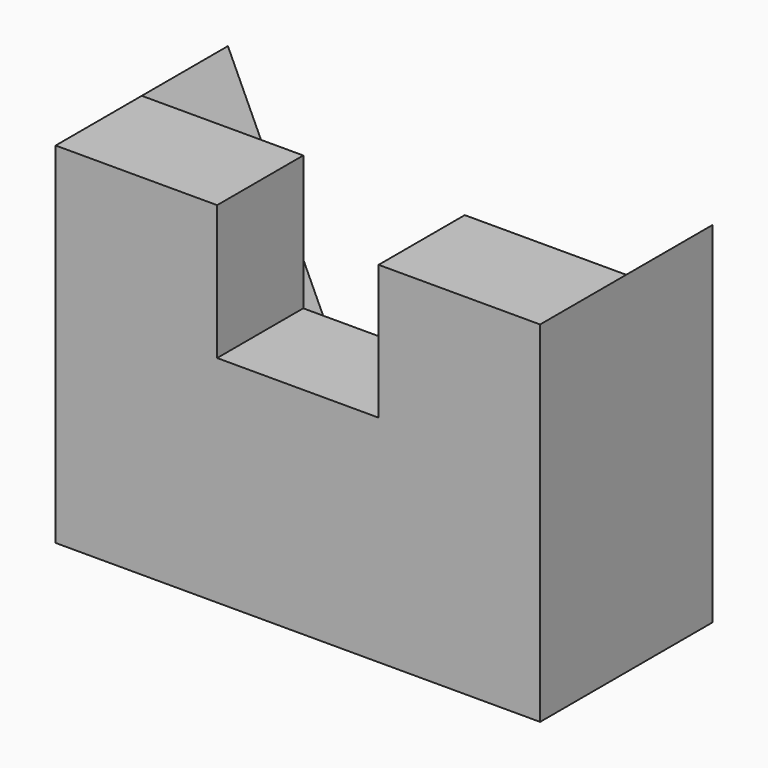
from build123d import *

# Parameters (mm, degrees)
F1_DEPTH = 20
F3_DEPTH = 20


# Not quite as in the source:
# - a feature names something its author has since deleted; it is built from what else it names


with BuildPart() as f1:
    # F0 (on Front) → F1 (new body)
    with BuildSketch(Plane.XZ):
        Polygon((-15, -32.5), (-45, 32.5), (-45, -32.5), align=None)
        Polygon((-15, 32.5), (-45, 32.5), (-15, -32.5), (15, -32.5), (45, 32.5), (15, 32.5), (15, 7.5), (-15, 7.5), align=None)
        Polygon((45, 32.5), (15, -32.5), (45, -32.5), align=None)
    extrude(amount=F1_DEPTH)

    # F0 (on Front) → F3 (join)
    with BuildSketch(Plane.XZ):
        Polygon((-15, -32.5), (-45, 32.5), (-45, -32.5), align=None)
        Polygon((45, 32.5), (15, -32.5), (45, -32.5), align=None)
    extrude(amount=-F3_DEPTH)


solid = f1.part
